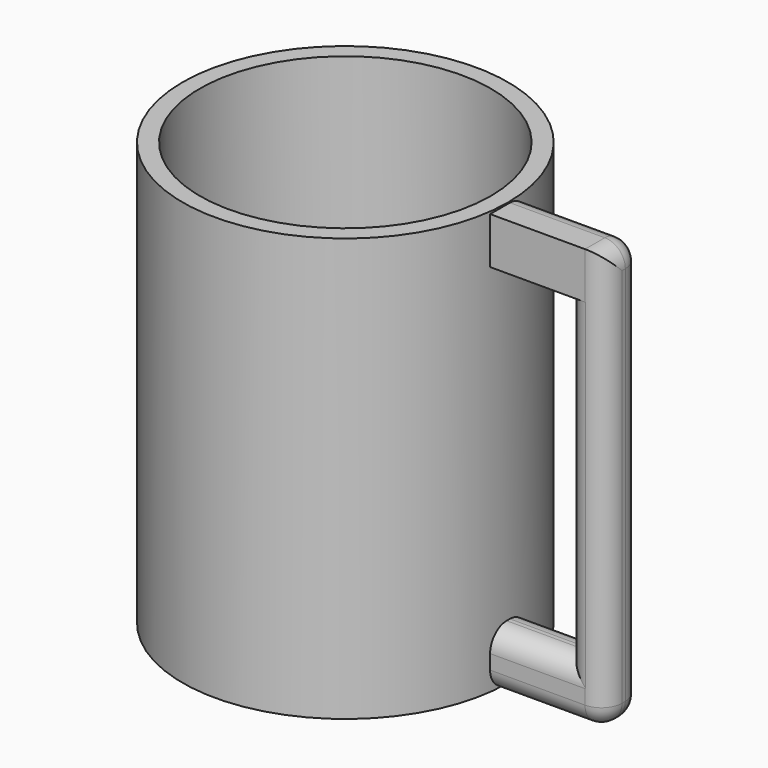
from build123d import *

# Parameters (mm, degrees)
F0_R         = 40.2600949405
F1_DEPTH     = 104.648
F2_R         = 35.9958099421
F3_DEPTH     = 97.536
F4_W         = 18.675433821
F4_H         = 79.0959624574
F5_DEPTH     = 5.588
F6_DEPTH     = 5.588
F7_DEPTH     = 72.39
F8_T1_DEPTH  = 18.796
F8_T3_DEPTH  = 1.016
F8_T5_DEPTH  = 31.375433821
F8_T7_DEPTH  = 79.0959624574
F8_T9_DEPTH  = 112.001993413
F8_T11_DEPTH = 94.221993413
F8_T13_DEPTH = 36.1824306416
F8_S17_W     = 5.08
F8_S17_H     = 5.08
F8_T18_DEPTH = 5.08
F8_S23_W     = 5.08
F8_S23_H     = 5.08
F8_T24_DEPTH = 5.08
F8_S29_W     = 5.08
F8_S29_H     = 5.08
F8_T30_DEPTH = 5.08
F8_T37_DEPTH = 44.075433821
F8_T41_DEPTH = 91.7959624574
F8_T48_DEPTH = 44.075433821
F8_T52_DEPTH = 91.7959624574
F8_T59_DEPTH = 91.7959624574
F8_T63_DEPTH = 44.075433821


# Not quite as in the source:
# - a fillet or chamfer that OpenCascade refuses, or shapes differently, is made with other operations: its cross-section is extruded or revolved along the edge and cut away or added


with BuildPart() as f1:
    # F0 (on Top) → F1 (new body)
    with BuildSketch(Plane.XY):
        with Locations((-39.6676883101, 0)):
            Circle(F0_R)
    extrude(amount=F1_DEPTH)

    # F2 (on face) → F3 (cut)
    with BuildSketch(Plane.XY.offset(104.648)):
        with Locations((-39.6676883101, 0)):
            Circle(F2_R)
    extrude(amount=-F3_DEPTH, mode=Mode.SUBTRACT)


with BuildPart() as f5:
    # F4 (on Front) → F5 (new body)
    with BuildSketch(Plane.XZ):
        Polygon((0.6275248015, 13.7512059882), (0.6275248015, 0), (29.1899554431, 0), (29.1899554431, 104.381993413), (0.6275248015, 104.381993413), (0.6275248015, 92.8471684456), (19.3029586226, 92.8471684456), (19.3029586226, 13.7512059882), align=None)
        with Locations((9.9652417121, 53.2991872169)):
            Rectangle(F4_W, F4_H)
    extrude(amount=F5_DEPTH)

    # F4 (on Front) → F6 (join)
    with BuildSketch(Plane.XZ):
        Polygon((0.6275248015, 13.7512059882), (0.6275248015, 0), (29.1899554431, 0), (29.1899554431, 104.381993413), (0.6275248015, 104.381993413), (0.6275248015, 92.8471684456), (19.3029586226, 92.8471684456), (19.3029586226, 13.7512059882), align=None)
    extrude(amount=-F6_DEPTH)

    # F4 (on Front) → F7 (cut)
    with BuildSketch(Plane.XZ):
        with Locations((9.9652417121, 53.2991872169)):
            Rectangle(F4_W, F4_H)
    extrude(amount=F7_DEPTH, mode=Mode.SUBTRACT)

    # F8: fillet of radius 5.08 on 12 edges, made by hand

    # F8_s2 → F8_t1 (cut)
    with BuildSketch(Plane.XZ.offset(-0.508)):
        with BuildLine():
            ThreePointArc((24.1099554431, 104.381993413), (27.7020578916, 102.8940958614), (29.1899554431, 99.301993413))
            Line((29.1899554431, 99.301993413), (29.1899554431, 104.381993413))
            Line((29.1899554431, 104.381993413), (24.1099554431, 104.381993413))
        make_face()
    extrude(amount=F8_T1_DEPTH, mode=Mode.SUBTRACT)

    # F8_s4 → F8_t3 (cut)
    with BuildSketch(Plane.XZ.offset(-0.508)):
        with BuildLine():
            ThreePointArc((24.1099554431, 0), (27.7020578916, 1.4878975516), (29.1899554431, 5.08))
            Line((29.1899554431, 5.08), (29.1899554431, 0))
            Line((29.1899554431, 0), (24.1099554431, 0))
        make_face()
    extrude(amount=F8_T3_DEPTH, mode=Mode.SUBTRACT)

    # F8_s6 → F8_t5 (cut)
    with BuildSketch(Plane.YZ.offset(-12.0724751985)):
        with BuildLine():
            ThreePointArc((-0.508, 13.7512059882), (-4.1001024484, 12.2633084367), (-5.588, 8.6712059882))
            Line((-5.588, 8.6712059882), (-5.588, 13.7512059882))
            Line((-5.588, 13.7512059882), (-0.508, 13.7512059882))
        make_face()
        with BuildLine():
            ThreePointArc((5.588, 97.9271684456), (4.1001024484, 94.3350659972), (0.508, 92.8471684456))
            Line((0.508, 92.8471684456), (5.588, 92.8471684456))
            Line((5.588, 92.8471684456), (5.588, 97.9271684456))
        make_face()
        with BuildLine():
            ThreePointArc((5.588, 8.6712059882), (4.1001024484, 12.2633084367), (0.508, 13.7512059882))
            Line((0.508, 13.7512059882), (5.588, 13.7512059882))
            Line((5.588, 13.7512059882), (5.588, 8.6712059882))
        make_face()
    extrude(amount=F8_T5_DEPTH, mode=Mode.SUBTRACT)

    # F8_s8 → F8_t7 (cut)
    with BuildSketch(Plane.XY.offset(13.7512059882)):
        with BuildLine():
            ThreePointArc((19.3029586226, -0.508), (20.7908561741, -4.1001024484), (24.3829586226, -5.588))
            Line((24.3829586226, -5.588), (19.3029586226, -5.588))
            Line((19.3029586226, -5.588), (19.3029586226, -0.508))
        make_face()
        with BuildLine():
            ThreePointArc((24.3829586226, 5.588), (20.7908561741, 4.1001024484), (19.3029586226, 0.508))
            Line((19.3029586226, 0.508), (19.3029586226, 5.588))
            Line((19.3029586226, 5.588), (24.3829586226, 5.588))
        make_face()
    extrude(amount=F8_T7_DEPTH, mode=Mode.SUBTRACT)

    # F8_s10 → F8_t9 (cut)
    with BuildSketch(Plane.XY.offset(5.08)):
        with BuildLine():
            ThreePointArc((29.1899554431, -0.508), (27.7020578916, -4.1001024484), (24.1099554431, -5.588))
            Line((24.1099554431, -5.588), (29.1899554431, -5.588))
            Line((29.1899554431, -5.588), (29.1899554431, -0.508))
        make_face()
    extrude(amount=F8_T9_DEPTH, mode=Mode.SUBTRACT)

    # F8_s12 → F8_t11 (cut)
    with BuildSketch(Plane.XY.offset(5.08)):
        with BuildLine():
            ThreePointArc((24.1099554431, 5.588), (27.7020578916, 4.1001024484), (29.1899554431, 0.508))
            Line((29.1899554431, 0.508), (29.1899554431, 5.588))
            Line((29.1899554431, 5.588), (24.1099554431, 5.588))
        make_face()
    extrude(amount=F8_T11_DEPTH, mode=Mode.SUBTRACT)

    # F8_s14 → F8_t13 (cut)
    with BuildSketch(Plane.YZ.offset(-12.0724751985)):
        with BuildLine():
            ThreePointArc((5.588, 99.301993413), (4.1001024484, 102.8940958614), (0.508, 104.381993413))
            Line((0.508, 104.381993413), (5.588, 104.381993413))
            Line((5.588, 104.381993413), (5.588, 99.301993413))
        make_face()
        with BuildLine():
            ThreePointArc((0.508, 0), (4.1001024484, 1.4878975516), (5.588, 5.08))
            Line((5.588, 5.08), (5.588, 0))
            Line((5.588, 0), (0.508, 0))
        make_face()
        with BuildLine():
            ThreePointArc((-0.508, 0), (-4.1001024484, 1.4878975516), (-5.588, 5.08))
            Line((-5.588, 5.08), (-5.588, 0))
            Line((-5.588, 0), (-0.508, 0))
        make_face()
    extrude(amount=F8_T13_DEPTH, mode=Mode.SUBTRACT)


with BuildPart() as f8_tool16:
    # F8_s17 → F8_t18 (new body)
    with BuildSketch(Plane.XZ.offset(-0.508)):
        with Locations((26.6499554431, 101.841993413)):
            Rectangle(F8_S17_W, F8_S17_H)
    extrude(amount=-F8_T18_DEPTH)

    # F8_s19 → F8_t20 (revolve, cut)
    with BuildSketch(Plane(origin=(24.1099554431, 0.508, 99.301993413), x_dir=(-0.7071067812, 0, -0.7071067812), z_dir=(0.7071067812, 0, -0.7071067812))):
        with BuildLine():
            ThreePointArc((0, -5.08), (5.08, 0), (0, 5.08))
            Line((0, 5.08), (0, -5.08))
        make_face()
    revolve(axis=Axis((24.1099554431, 0.508, 99.301993413), (0, 1, 0)), mode=Mode.SUBTRACT)


with BuildPart() as f5_1:
    add(f5.part)

    # F8_t15: cut F8_tool16
    add(f8_tool16.part, mode=Mode.SUBTRACT)


with BuildPart() as f8_tool22:
    # F8_s23 → F8_t24 (new body)
    with BuildSketch(Plane.XY.offset(5.08)):
        with Locations((26.6499554431, 3.048)):
            Rectangle(F8_S23_W, F8_S23_H)
    extrude(amount=-F8_T24_DEPTH)

    # F8_s25 → F8_t26 (revolve, cut)
    with BuildSketch(Plane(origin=(24.1099554431, 0.508, 5.08), x_dir=(-0.7071067812, -0.7071067812, 0), z_dir=(0.7071067812, -0.7071067812, 0))):
        with BuildLine():
            ThreePointArc((0, -5.08), (5.08, 0), (0, 5.08))
            Line((0, 5.08), (0, -5.08))
        make_face()
    revolve(axis=Axis((24.1099554431, 0.508, 5.08), (0, 0, -1)), mode=Mode.SUBTRACT)


with BuildPart() as f5_2:
    add(f5_1.part)

    # F8_t21: cut F8_tool22
    add(f8_tool22.part, mode=Mode.SUBTRACT)


with BuildPart() as f8_tool28:
    # F8_s29 → F8_t30 (new body)
    with BuildSketch(Plane.XY.offset(5.08)):
        with Locations((26.6499554431, -3.048)):
            Rectangle(F8_S29_W, F8_S29_H)
    extrude(amount=-F8_T30_DEPTH)

    # F8_s31 → F8_t32 (revolve, cut)
    with BuildSketch(Plane(origin=(24.1099554431, -0.508, 5.08), x_dir=(-0.7071067812, 0.7071067812, 0), z_dir=(-0.7071067812, -0.7071067812, 0))):
        with BuildLine():
            ThreePointArc((0, -5.08), (5.08, 0), (0, 5.08))
            Line((0, 5.08), (0, -5.08))
        make_face()
    revolve(axis=Axis((24.1099554431, -0.508, 5.08), (0, 0, -1)), mode=Mode.SUBTRACT)


with BuildPart() as f5_3:
    add(f5_2.part)

    # F8_t27: cut F8_tool28
    add(f8_tool28.part, mode=Mode.SUBTRACT)


with BuildPart() as f8_tool35:
    # F8_s36 → F8_t37 (new body)
    with BuildSketch(Plane.YZ.offset(32.0029586226)):
        with BuildLine():
            ThreePointArc((-0.508, 13.7512059882), (-4.1001024484, 12.2633084367), (-5.588, 8.6712059882))
            Line((-5.588, 8.6712059882), (-5.588, 13.7512059882))
            Line((-5.588, 13.7512059882), (-0.508, 13.7512059882))
        make_face()
    extrude(amount=-F8_T37_DEPTH)

    split(bisect_by=Plane.YZ.offset(19.3029586226), keep=Keep.TOP)


with BuildPart() as f8_tool39:
    # F8_s40 → F8_t41 (new body)
    with BuildSketch(Plane.XY.offset(92.8471684456)):
        with BuildLine():
            ThreePointArc((19.3029586226, -0.508), (20.7908561741, -4.1001024484), (24.3829586226, -5.588))
            Line((24.3829586226, -5.588), (19.3029586226, -5.588))
            Line((19.3029586226, -5.588), (19.3029586226, -0.508))
        make_face()
    extrude(amount=-F8_T41_DEPTH)

    split(bisect_by=Plane.XY.offset(13.7512059882), keep=Keep.BOTTOM)


with BuildPart() as f8_tool35_1:
    add(f8_tool35.part)

    # F8_t43: intersect F8_tool39
    add(f8_tool39.part, mode=Mode.INTERSECT)


with BuildPart() as f5_4:
    add(f5_3.part)

    # F8_t33: cut F8_tool35
    add(f8_tool35_1.part, mode=Mode.SUBTRACT)


with BuildPart() as f8_tool46:
    # F8_s47 → F8_t48 (new body)
    with BuildSketch(Plane.YZ.offset(-12.0724751985)):
        with BuildLine():
            ThreePointArc((5.588, 97.9271684456), (4.1001024484, 94.3350659972), (0.508, 92.8471684456))
            Line((0.508, 92.8471684456), (5.588, 92.8471684456))
            Line((5.588, 92.8471684456), (5.588, 97.9271684456))
        make_face()
    extrude(amount=F8_T48_DEPTH)

    split(bisect_by=Plane.YZ.offset(19.3029586226), keep=Keep.TOP)


with BuildPart() as f8_tool50:
    # F8_s51 → F8_t52 (new body)
    with BuildSketch(Plane.XY.offset(105.5471684456)):
        with BuildLine():
            ThreePointArc((24.3829586226, 5.588), (20.7908561741, 4.1001024484), (19.3029586226, 0.508))
            Line((19.3029586226, 0.508), (19.3029586226, 5.588))
            Line((19.3029586226, 5.588), (24.3829586226, 5.588))
        make_face()
    extrude(amount=-F8_T52_DEPTH)

    split(bisect_by=Plane.XY.offset(92.8471684456), keep=Keep.TOP)


with BuildPart() as f8_tool46_1:
    add(f8_tool46.part)

    # F8_t54: intersect F8_tool50
    add(f8_tool50.part, mode=Mode.INTERSECT)


with BuildPart() as f5_5:
    add(f5_4.part)

    # F8_t44: cut F8_tool46
    add(f8_tool46_1.part, mode=Mode.SUBTRACT)


with BuildPart() as f8_tool57:
    # F8_s58 → F8_t59 (new body)
    with BuildSketch(Plane.XY.offset(92.8471684456)):
        with BuildLine():
            ThreePointArc((24.3829586226, 5.588), (20.7908561741, 4.1001024484), (19.3029586226, 0.508))
            Line((19.3029586226, 0.508), (19.3029586226, 5.588))
            Line((19.3029586226, 5.588), (24.3829586226, 5.588))
        make_face()
    extrude(amount=-F8_T59_DEPTH)

    split(bisect_by=Plane.XY.offset(13.7512059882), keep=Keep.BOTTOM)


with BuildPart() as f8_tool61:
    # F8_s62 → F8_t63 (new body)
    with BuildSketch(Plane.YZ.offset(32.0029586226)):
        with BuildLine():
            ThreePointArc((5.588, 8.6712059882), (4.1001024484, 12.2633084367), (0.508, 13.7512059882))
            Line((0.508, 13.7512059882), (5.588, 13.7512059882))
            Line((5.588, 13.7512059882), (5.588, 8.6712059882))
        make_face()
    extrude(amount=-F8_T63_DEPTH)

    split(bisect_by=Plane.YZ.offset(19.3029586226), keep=Keep.TOP)


with BuildPart() as f8_tool57_1:
    add(f8_tool57.part)

    # F8_t65: intersect F8_tool61
    add(f8_tool61.part, mode=Mode.INTERSECT)


with BuildPart() as f5_6:
    add(f5_5.part)

    # F8_t55: cut F8_tool57
    add(f8_tool57_1.part, mode=Mode.SUBTRACT)


solid = Compound([f1.part, f5_6.part])
